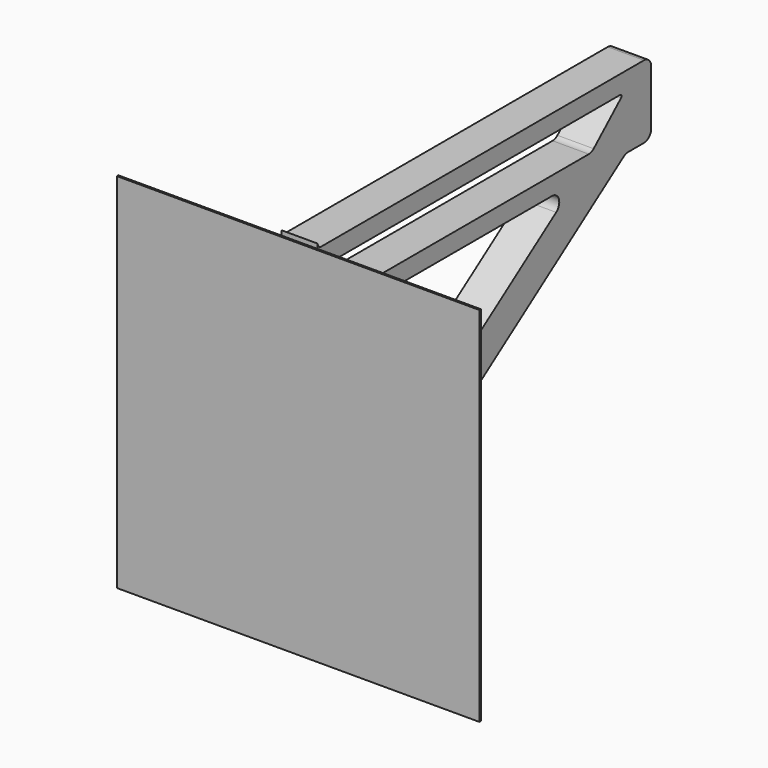
from build123d import *

# Parameters (mm, degrees)
F4_DEPTH = 5
F0_W     = 100
F0_H     = 100
F6_DEPTH = 0.5


# Not quite as in the source:
# - the program builds the solid bodies; features that only make, move or delete a surface that nothing else refers to are left out


with BuildPart() as f4:
    # F1 (on Right) → F4 (new body, symmetric)
    with BuildSketch(Plane.YZ):
        with BuildLine():
            ThreePointArc((104.2533004827, 45), (104.7201177173, 44.6791135659), (104.5877536809, 44.128326678))
            Line((104.5877536809, 44.128326678), (95.1566060497, 35.6416333901))
            ThreePointArc((95.1566060497, 35.6416333901), (94.3799078888, 35.1659138271), (93.4843400592, 35))
            Line((93.4843400592, 35), (5, 35))
            ThreePointArc((5, 35), (1.4698085841, 36.4591316648), (2.27993e-05, 39.9849005732))
            Line((2.27993e-05, 39.9849005732), (0.0226491659, 25.0000171511))
            ThreePointArc((0.0226491659, 25.0000171511), (1.4871213238, 28.5355399698), (5.0226491659, 30))
            Line((5.0226491659, 30), (80.7907660618, 30))
            ThreePointArc((80.7907660618, 30), (83.1753398645, 28.2508713467), (82.2231725759, 25.4510462235))
            Line((82.2231725759, 25.4510462235), (3.7000322722, -29.44382694))
            ThreePointArc((3.7000322722, -29.44382694), (1.3024238225, -29.6010647183), (0.0526297849, -27.5489280609))
            Line((0.0526297849, -27.5489280609), (0.0953742048, -45.3789287217))
            ThreePointArc((0.0953742048, -45.3789287217), (0.3564868473, -44.3043555559), (1.0855882207, -43.4729119391))
            Line((1.0855882207, -43.4729119391), (105.5380785244, 29.5489537765))
            ThreePointArc((105.5380785244, 29.5489537765), (106.2196136918, 29.8845738027), (106.9704850386, 30))
            Line((106.9704850386, 30), (112.5, 30))
            ThreePointArc((112.5, 30), (114.267766953, 30.732233047), (115, 32.5))
            Line((115, 32.5), (115, 47.5574878287))
            ThreePointArc((115, 47.5574878287), (114.267766953, 49.3252547817), (112.5, 50.0574878287))
            Line((112.5, 50.0574878287), (1.2462358677, 50.0574878287))
            ThreePointArc((1.2462358677, 50.0574878287), (0.3800812524, 50.4162608175), (0.0213082636, 51.2824154329))
            Line((0.0213082636, 51.2824154329), (3.5669e-05, 40.018886193))
            ThreePointArc((3.5669e-05, 40.018886193), (1.471149689, 43.54220489), (5, 45))
            Line((5, 45), (104.2533004827, 45))
        make_face()
    extrude(amount=F4_DEPTH, both=True)


with BuildPart() as f6:
    # F0 (on Front) → F6 (new body)
    with BuildSketch(Plane.XZ):
        Rectangle(F0_W, F0_H)
    extrude(amount=F6_DEPTH)


solid = Compound([f4.part, f6.part])
